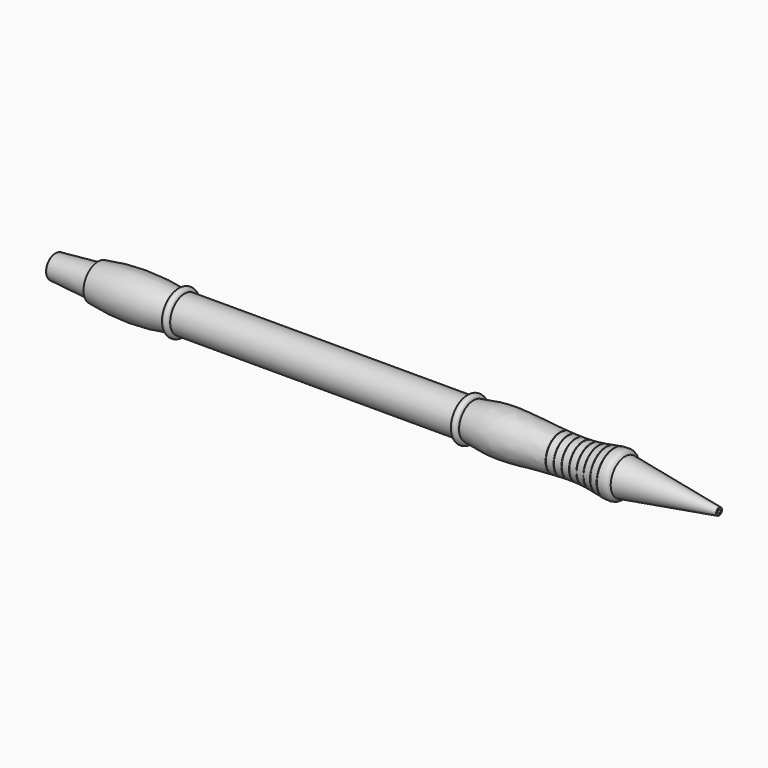
from build123d import *

# Parameters (mm, degrees)
F0_W     = 61.9125
F0_H     = 3.96875
F2_R     = 0.396875
F3_DEPTH = 127
F5_DEPTH = 6.35


# Not quite as in the source:
# - a length typed as a fraction of an inch, garbled in the dataset ("3 / 203.2 mm" for 3/8 in), is restored


with BuildPart() as f1:
    # F0 (on Front) → F1 (revolve)
    with BuildSketch(Plane.XZ):
        Polygon((-20.6375, 0), (0, 0), (0, 0.79375), (-20.6375, 3.96875), (-20.6375, 3.86953125), align=None)
        with BuildLine():
            Line((-55.5625, 0), (-20.6375, 0))
            Line((-20.6375, 0), (-20.6375, 3.86953125))
            add(Edge.make_bspline(
                [(-23.01875, 4.6666390523), (-22.3334209886, 4.7571479317), (-21.1593030797, 4.80554296), (-20.820641756, 4.1980514041), (-20.6375, 3.86953125)],
                knots=[0.8176786656, 0.8176786656, 0.8176786656, 0.8176786656, 0.9014040075, 1, 1, 1, 1], degree=3))
            add(Edge.make_bspline(
                [(-23.11796875, 4.6532074188), (-23.0845644542, 4.6578353858), (-23.0514904461, 4.6623151422), (-23.01875, 4.6666390523)],
                knots=[0.8136788276, 0.8136788276, 0.8136788276, 0.8136788276, 0.8176786656, 0.8176786656, 0.8176786656, 0.8176786656], degree=3))
            add(Edge.make_bspline(
                [(-24.70546875, 4.3927589159), (-24.117599982, 4.4946500328), (-23.585442034, 4.5884417681), (-23.11796875, 4.6532074188)],
                knots=[0.7577034694, 0.7577034694, 0.7577034694, 0.7577034694, 0.8136788276, 0.8136788276, 0.8136788276, 0.8136788276], degree=3))
            add(Edge.make_bspline(
                [(-24.8046875, 4.3755800551), (-24.7714411529, 4.381329263), (-24.7383677119, 4.3870567725), (-24.70546875, 4.3927589159)],
                knots=[0.7545709145, 0.7545709145, 0.7545709145, 0.7545709145, 0.7577034694, 0.7577034694, 0.7577034694, 0.7577034694], degree=3))
            add(Edge.make_bspline(
                [(-26.3921875, 4.1175295828), (-25.8284362948, 4.2003483086), (-25.2975614293, 4.290348595), (-24.8046875, 4.3755800551)],
                knots=[0.7081310867, 0.7081310867, 0.7081310867, 0.7081310867, 0.7545709145, 0.7545709145, 0.7545709145, 0.7545709145], degree=3))
            add(Edge.make_bspline(
                [(-26.49140625, 4.1030791182), (-26.4582216318, 4.107869798), (-26.4251483737, 4.1126874157), (-26.3921875, 4.1175295828)],
                knots=[0.7054158867, 0.7054158867, 0.7054158867, 0.7054158867, 0.7081310867, 0.7081310867, 0.7081310867, 0.7081310867], degree=3))
            add(Edge.make_bspline(
                [(-28.07890625, 3.911617905), (-27.5263903446, 3.9636105229), (-26.9960232193, 4.0302303565), (-26.49140625, 4.1030791182)],
                knots=[0.6641276004, 0.6641276004, 0.6641276004, 0.6641276004, 0.7054158867, 0.7054158867, 0.7054158867, 0.7054158867], degree=3))
            add(Edge.make_bspline(
                [(-28.178125, 3.9024617612), (-28.1449736113, 3.9054604557), (-28.111900439, 3.9085130998), (-28.07890625, 3.911617905)],
                knots=[0.6616620179, 0.6616620179, 0.6616620179, 0.6616620179, 0.6641276004, 0.6641276004, 0.6641276004, 0.6641276004], degree=3))
            add(Edge.make_bspline(
                [(-29.765625, 3.8050576904), (-29.3599047919, 3.8191656206), (-28.8256037638, 3.8476182782), (-28.3092095533, 3.8906045646), (-28.178125, 3.9024617612)],
                knots=[0.6236109964, 0.6236109964, 0.6236109964, 0.6236109964, 0.6519128102, 0.6616620179, 0.6616620179, 0.6616620179, 0.6616620179], degree=3))
            add(Edge.make_bspline(
                [(-29.86484375, 3.8017529539), (-29.8317163379, 3.8028081635), (-29.7986431352, 3.8039095653), (-29.765625, 3.8050576904)],
                knots=[0.6213077512, 0.6213077512, 0.6213077512, 0.6213077512, 0.6236109964, 0.6236109964, 0.6236109964, 0.6236109964], degree=3))
            add(Edge.make_bspline(
                [(-31.45234375, 3.784082632), (-30.9121459933, 3.7800664759), (-30.3818920053, 3.7852833825), (-29.86484375, 3.8017529539)],
                knots=[0.5853590058, 0.5853590058, 0.5853590058, 0.5853590058, 0.6213077512, 0.6213077512, 0.6213077512, 0.6213077512], degree=3))
            add(Edge.make_bspline(
                [(-31.5515625, 3.7849225925), (-31.5184528913, 3.7846083822), (-31.4853797259, 3.7843282414), (-31.45234375, 3.784082632)],
                knots=[0.5831605481, 0.5831605481, 0.5831605481, 0.5831605481, 0.5853590058, 0.5853590058, 0.5853590058, 0.5853590058], degree=3))
            add(Edge.make_bspline(
                [(-33.1390625, 3.8232760222), (-32.6028075002, 3.8032526962), (-32.0726712529, 3.7898679164), (-31.5515625, 3.7849225925)],
                knots=[0.5485592476, 0.5485592476, 0.5485592476, 0.5485592476, 0.5831605481, 0.5831605481, 0.5831605481, 0.5831605481], degree=3))
            add(Edge.make_bspline(
                [(-33.23828125, 3.8270534172), (-33.205185546, 3.8257693509), (-33.1721124023, 3.8245100787), (-33.1390625, 3.8232760222)],
                knots=[0.5464267368, 0.5464267368, 0.5464267368, 0.5464267368, 0.5485592476, 0.5485592476, 0.5485592476, 0.5485592476], degree=3))
            add(Edge.make_bspline(
                [(-34.82578125, 3.9050898088), (-34.2927563116, 3.8739707874), (-33.7626866879, 3.8473996028), (-33.23828125, 3.8270534172)],
                knots=[0.5126368442, 0.5126368442, 0.5126368442, 0.5126368442, 0.5464267368, 0.5464267368, 0.5464267368, 0.5464267368], degree=3))
            add(Edge.make_bspline(
                [(-34.925, 3.9109325272), (-34.8919161443, 3.9089677243), (-34.8588430121, 3.9070200181), (-34.82578125, 3.9050898088)],
                knots=[0.5105409697, 0.5105409697, 0.5105409697, 0.5105409697, 0.5126368442, 0.5126368442, 0.5126368442, 0.5126368442], degree=3))
            Line((-34.925, 3.9109325272), (-34.925, 4.0101512772))
            add(Edge.make_bspline(
                [(-53.975, 3.96875), (-51.6734572333, 4.3916770235), (-47.2028394574, 5.2131890531), (-38.8351054319, 4.2423668511), (-34.925, 4.0101512772)],
                knots=[0, 0, 0, 0, 0.2628343408, 0.5105409697, 0.5105409697, 0.5105409697, 0.5105409697], degree=3))
            ThreePointArc((-53.975, 3.96875), (-54.76875, 4.7625), (-55.5625, 3.96875))
            Line((-55.5625, 3.96875), (-55.5625, 0))
        make_face()
        with Locations((-86.51875, 1.984375)):
            Rectangle(F0_W, F0_H)
        with BuildLine():
            add(Edge.make_bspline(
                [(-23.01875, 4.6666390523), (-22.3334209886, 4.7571479317), (-21.1593030797, 4.80554296), (-20.820641756, 4.1980514041), (-20.6375, 3.86953125)],
                knots=[0.8176786656, 0.8176786656, 0.8176786656, 0.8176786656, 0.9014040075, 1, 1, 1, 1], degree=3))
            Line((-20.6375, 3.86953125), (-20.6375, 3.96875))
            add(Edge.make_bspline(
                [(-23.01875, 4.7658578023), (-22.3334209886, 4.8563666817), (-21.1593030797, 4.90476171), (-20.820641756, 4.2972701541), (-20.6375, 3.96875)],
                knots=[0.8176786656, 0.8176786656, 0.8176786656, 0.8176786656, 0.9014040075, 1, 1, 1, 1], degree=3))
            Line((-23.01875, 4.7658578023), (-23.01875, 4.6666390523))
        make_face()
        with BuildLine():
            Line((-136.525, 0), (-117.475, 0))
            Line((-117.475, 0), (-117.475, 3.96875))
            ThreePointArc((-117.475, 3.96875), (-118.26875, 4.7625), (-119.0625, 3.96875))
            ThreePointArc((-119.0625, 3.96875), (-127.79375, 4.7625004164), (-136.525, 3.96875))
            Line((-136.525, 3.96875), (-136.525, 3.3734375))
            Line((-136.525, 3.3734375), (-136.525, 0))
        make_face()
        with BuildLine():
            Line((-146.05, 0), (-136.525, 0))
            Line((-136.525, 0), (-136.525, 3.3734375))
            Line((-136.525, 3.3734375), (-145.6860836748, 2.6100138604))
            ThreePointArc((-145.6860836748, 2.6100138604), (-145.9451782825, 2.4832375911), (-146.05, 2.2145097626))
            Line((-146.05, 2.2145097626), (-146.05, 0))
        make_face()
        with BuildLine():
            add(Edge.make_bspline(
                [(-24.70546875, 4.3927589159), (-24.117599982, 4.4946500328), (-23.585442034, 4.5884417681), (-23.11796875, 4.6532074188)],
                knots=[0.7577034694, 0.7577034694, 0.7577034694, 0.7577034694, 0.8136788276, 0.8136788276, 0.8136788276, 0.8136788276], degree=3))
            Line((-23.11796875, 4.6532074188), (-23.11796875, 4.7524261688))
            add(Edge.make_bspline(
                [(-24.70546875, 4.4919776659), (-24.117599982, 4.5938687828), (-23.585442034, 4.6876605181), (-23.11796875, 4.7524261688)],
                knots=[0.7577034694, 0.7577034694, 0.7577034694, 0.7577034694, 0.8136788276, 0.8136788276, 0.8136788276, 0.8136788276], degree=3))
            Line((-24.70546875, 4.4919776659), (-24.70546875, 4.3927589159))
        make_face()
        with BuildLine():
            add(Edge.make_bspline(
                [(-34.82578125, 4.0043085588), (-34.2927563116, 3.9731895374), (-33.7626866879, 3.9466183528), (-33.23828125, 3.9262721672)],
                knots=[0.5126368442, 0.5126368442, 0.5126368442, 0.5126368442, 0.5464267368, 0.5464267368, 0.5464267368, 0.5464267368], degree=3))
            Line((-34.82578125, 4.0043085588), (-34.82578125, 3.9050898088))
            add(Edge.make_bspline(
                [(-34.82578125, 3.9050898088), (-34.2927563116, 3.8739707874), (-33.7626866879, 3.8473996028), (-33.23828125, 3.8270534172)],
                knots=[0.5126368442, 0.5126368442, 0.5126368442, 0.5126368442, 0.5464267368, 0.5464267368, 0.5464267368, 0.5464267368], degree=3))
            Line((-33.23828125, 3.8270534172), (-33.23828125, 3.9262721672))
        make_face()
        with BuildLine():
            add(Edge.make_bspline(
                [(-26.3921875, 4.1175295828), (-25.8284362948, 4.2003483086), (-25.2975614293, 4.290348595), (-24.8046875, 4.3755800551)],
                knots=[0.7081310867, 0.7081310867, 0.7081310867, 0.7081310867, 0.7545709145, 0.7545709145, 0.7545709145, 0.7545709145], degree=3))
            Line((-24.8046875, 4.3755800551), (-24.8046875, 4.4747988051))
            add(Edge.make_bspline(
                [(-26.3921875, 4.2167483328), (-25.8284362948, 4.2995670586), (-25.2975614293, 4.389567345), (-24.8046875, 4.4747988051)],
                knots=[0.7081310867, 0.7081310867, 0.7081310867, 0.7081310867, 0.7545709145, 0.7545709145, 0.7545709145, 0.7545709145], degree=3))
            Line((-26.3921875, 4.2167483328), (-26.3921875, 4.1175295828))
        make_face()
        with BuildLine():
            add(Edge.make_bspline(
                [(-33.1390625, 3.9224947722), (-32.6028075002, 3.9024714462), (-32.0726712529, 3.8890866664), (-31.5515625, 3.8841413425)],
                knots=[0.5485592476, 0.5485592476, 0.5485592476, 0.5485592476, 0.5831605481, 0.5831605481, 0.5831605481, 0.5831605481], degree=3))
            Line((-33.1390625, 3.9224947722), (-33.1390625, 3.8232760222))
            add(Edge.make_bspline(
                [(-33.1390625, 3.8232760222), (-32.6028075002, 3.8032526962), (-32.0726712529, 3.7898679164), (-31.5515625, 3.7849225925)],
                knots=[0.5485592476, 0.5485592476, 0.5485592476, 0.5485592476, 0.5831605481, 0.5831605481, 0.5831605481, 0.5831605481], degree=3))
            Line((-31.5515625, 3.7849225925), (-31.5515625, 3.8841413425))
        make_face()
        with BuildLine():
            add(Edge.make_bspline(
                [(-28.07890625, 3.911617905), (-27.5263903446, 3.9636105229), (-26.9960232193, 4.0302303565), (-26.49140625, 4.1030791182)],
                knots=[0.6641276004, 0.6641276004, 0.6641276004, 0.6641276004, 0.7054158867, 0.7054158867, 0.7054158867, 0.7054158867], degree=3))
            Line((-26.49140625, 4.1030791182), (-26.49140625, 4.2022978682))
            add(Edge.make_bspline(
                [(-28.07890625, 4.010836655), (-27.5263903446, 4.0628292729), (-26.9960232193, 4.1294491065), (-26.49140625, 4.2022978682)],
                knots=[0.6641276004, 0.6641276004, 0.6641276004, 0.6641276004, 0.7054158867, 0.7054158867, 0.7054158867, 0.7054158867], degree=3))
            Line((-28.07890625, 4.010836655), (-28.07890625, 3.911617905))
        make_face()
        with BuildLine():
            add(Edge.make_bspline(
                [(-31.45234375, 3.883301382), (-30.9121459933, 3.8792852259), (-30.3818920053, 3.8845021325), (-29.86484375, 3.9009717039)],
                knots=[0.5853590058, 0.5853590058, 0.5853590058, 0.5853590058, 0.6213077512, 0.6213077512, 0.6213077512, 0.6213077512], degree=3))
            Line((-31.45234375, 3.883301382), (-31.45234375, 3.784082632))
            add(Edge.make_bspline(
                [(-31.45234375, 3.784082632), (-30.9121459933, 3.7800664759), (-30.3818920053, 3.7852833825), (-29.86484375, 3.8017529539)],
                knots=[0.5853590058, 0.5853590058, 0.5853590058, 0.5853590058, 0.6213077512, 0.6213077512, 0.6213077512, 0.6213077512], degree=3))
            Line((-29.86484375, 3.8017529539), (-29.86484375, 3.9009717039))
        make_face()
        with BuildLine():
            add(Edge.make_bspline(
                [(-29.765625, 3.8050576904), (-29.3599047919, 3.8191656206), (-28.8256037638, 3.8476182782), (-28.3092095533, 3.8906045646), (-28.178125, 3.9024617612)],
                knots=[0.6236109964, 0.6236109964, 0.6236109964, 0.6236109964, 0.6519128102, 0.6616620179, 0.6616620179, 0.6616620179, 0.6616620179], degree=3))
            Line((-28.178125, 3.9024617612), (-28.178125, 4.0016805112))
            add(Edge.make_bspline(
                [(-29.765625, 3.9042764404), (-29.3599047919, 3.9183843706), (-28.8256037638, 3.9468370282), (-28.3092095533, 3.9898233146), (-28.178125, 4.0016805112)],
                knots=[0.6236109964, 0.6236109964, 0.6236109964, 0.6236109964, 0.6519128102, 0.6616620179, 0.6616620179, 0.6616620179, 0.6616620179], degree=3))
            Line((-29.765625, 3.9042764404), (-29.765625, 3.8050576904))
        make_face()
    revolve(axis=Axis((-73.025, 0, 0), (-1, 0, 0)))

    # F2 (on face) → F3 (cut)
    with BuildSketch(Plane.YZ):
        Circle(F2_R)
    extrude(amount=-F3_DEPTH, mode=Mode.SUBTRACT)

    # F4 (on face) → F5 (cut)
    with BuildSketch(Plane(origin=(-146.05, 0, 0), x_dir=(0, -1, 0), z_dir=(-1, 0, 0))):
        with BuildLine():
            Line((-0.396875, 0.6874076643), (-0.396875, 1.5370902655))
            ThreePointArc((-0.396875, 1.5370902655), (-1.3748153285, 0.79375), (-1.5295967179, -0.4248413006))
            Line((-1.5295967179, -0.4248413006), (-0.79375, 0))
            ThreePointArc((-0.79375, 0), (-0.6874076643, 0.396875), (-0.396875, 0.6874076643))
        make_face()
        with BuildLine():
            ThreePointArc((1.5295967179, -0.4248413006), (1.5729575709, -0.2143845382), (1.5875, 0))
            ThreePointArc((1.5875, 0), (1.2550289464, 0.9721412417), (0.396875, 1.5370902655))
            Line((0.396875, 1.5370902655), (0.396875, 0.6874076643))
            ThreePointArc((0.396875, 0.6874076643), (0.6874076643, 0.396875), (0.79375, 0))
            Line((0.79375, 0), (1.5295967179, -0.4248413006))
        make_face()
        with BuildLine():
            ThreePointArc((-1.1327217179, -1.1122489649), (0, -1.5875), (1.1327217179, -1.1122489649))
            Line((1.1327217179, -1.1122489649), (0.396875, -0.6874076643))
            ThreePointArc((0.396875, -0.6874076643), (0, -0.79375), (-0.396875, -0.6874076643))
            Line((-0.396875, -0.6874076643), (-1.1327217179, -1.1122489649))
        make_face()
    extrude(amount=-F5_DEPTH, mode=Mode.SUBTRACT)


solid = f1.part
